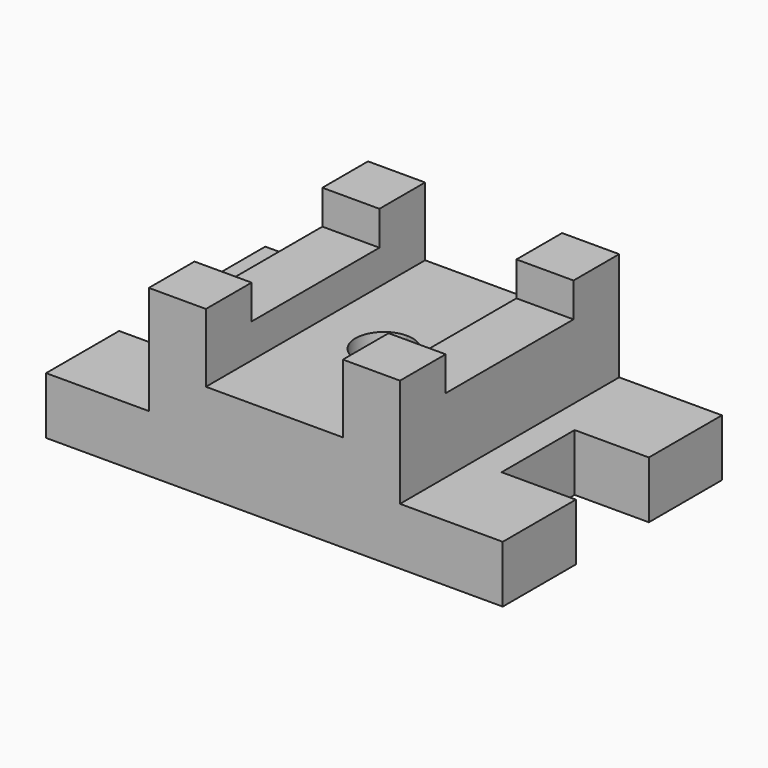
from build123d import *

# Parameters (mm, degrees)
F0_W     = 31.75
F0_H     = 88.9
F0_H_2   = 31.75
F1_DEPTH = 31.75
F2_DEPTH = 31.751
F3_DEPTH = 31.751
F4_DEPTH = 22.225
F5_DEPTH = 60.325
F6_DEPTH = 41.275
F7_SCALE = 0.5


with BuildPart() as f1:
    # F0 (on Top) → F1 (new body)
    with BuildSketch(Plane.XY):
        Polygon((-69.85, 44.45), (-69.85, 76.2), (-127, 76.2), (-127, 25.4), (-85.725, 25.4), (-85.725, -25.4), (-127, -25.4), (-127, -76.2), (-69.85, -76.2), (-69.85, -44.45), align=None)
        Polygon((-85.725, 25.4), (-127, 25.4), (-127, 0), (-127, -25.4), (-85.725, -25.4), align=None)
        with Locations((-53.975, 0)):
            Rectangle(F0_W, F0_H)
        with Locations((-53.975, 60.325)):
            Rectangle(F0_W, F0_H_2)
        with Locations((-53.975, -60.325)):
            Rectangle(F0_W, F0_H_2)
        with BuildLine():
            ThreePointArc((0, -15.875), (-15.875, 0), (0, 15.875))
            Line((0, 15.875), (0, 76.2))
            Line((0, 76.2), (-38.1, 76.2))
            Line((-38.1, 76.2), (-38.1, 44.45))
            Line((-38.1, 44.45), (-38.1, -44.45))
            Line((-38.1, -44.45), (-38.1, -76.2))
            Line((-38.1, -76.2), (0, -76.2))
            Line((0, -76.2), (0, -15.875))
        make_face()
        with BuildLine():
            Line((0, -15.875), (0, 0))
            Line((0, 0), (0, 15.875))
            ThreePointArc((0, 15.875), (-15.875, 0), (0, -15.875))
        make_face()
        with BuildLine():
            Line((0, 76.2), (0, 15.875))
            ThreePointArc((0, 15.875), (11.22532, 11.22532), (15.875, 0))
            ThreePointArc((15.875, 0), (11.22532, -11.22532), (0, -15.875))
            Line((0, -15.875), (0, -76.2))
            Line((0, -76.2), (38.1, -76.2))
            Line((38.1, -76.2), (38.1, -44.45))
            Line((38.1, -44.45), (38.1, 44.45))
            Line((38.1, 44.45), (38.1, 76.2))
            Line((38.1, 76.2), (0, 76.2))
        make_face()
        with BuildLine():
            Line((0, 15.875), (0, 0))
            Line((0, 0), (0, -15.875))
            ThreePointArc((0, -15.875), (11.22532, -11.22532), (15.875, 0))
            ThreePointArc((15.875, 0), (11.22532, 11.22532), (0, 15.875))
        make_face()
        with Locations((53.975, 0)):
            Rectangle(F0_W, F0_H)
        with Locations((53.975, 60.325)):
            Rectangle(F0_W, F0_H_2)
        with Locations((53.975, -60.325)):
            Rectangle(F0_W, F0_H_2)
        Polygon((127, 76.2), (69.85, 76.2), (69.85, 44.45), (69.85, -44.45), (69.85, -76.2), (127, -76.2), (127, -25.4), (85.725, -25.4), (85.725, 25.4), (127, 25.4), align=None)
        Polygon((127, 0), (127, 25.4), (85.725, 25.4), (85.725, -25.4), (127, -25.4), align=None)
    extrude(amount=-F1_DEPTH)

    # F0 (on Top) → F2 (cut, through all)
    with BuildSketch(Plane.XY):
        Polygon((-85.725, 25.4), (-127, 25.4), (-127, 0), (-127, -25.4), (-85.725, -25.4), align=None)
        Polygon((127, 0), (127, 25.4), (85.725, 25.4), (85.725, -25.4), (127, -25.4), align=None)
    extrude(amount=-F2_DEPTH, mode=Mode.SUBTRACT)

    # F0 (on Top) → F3 (cut, through all)
    with BuildSketch(Plane.XY):
        with BuildLine():
            Line((0, 15.875), (0, 0))
            Line((0, 0), (0, -15.875))
            ThreePointArc((0, -15.875), (11.22532, -11.22532), (15.875, 0))
            ThreePointArc((15.875, 0), (11.22532, 11.22532), (0, 15.875))
        make_face()
        with BuildLine():
            Line((0, -15.875), (0, 0))
            Line((0, 0), (0, 15.875))
            ThreePointArc((0, 15.875), (-15.875, 0), (0, -15.875))
        make_face()
    extrude(amount=-F3_DEPTH, mode=Mode.SUBTRACT)

    # F0 (on Top) → F4 (join)
    with BuildSketch(Plane.XY):
        with BuildLine():
            ThreePointArc((0, -15.875), (-15.875, 0), (0, 15.875))
            Line((0, 15.875), (0, 76.2))
            Line((0, 76.2), (-38.1, 76.2))
            Line((-38.1, 76.2), (-38.1, 44.45))
            Line((-38.1, 44.45), (-38.1, -44.45))
            Line((-38.1, -44.45), (-38.1, -76.2))
            Line((-38.1, -76.2), (0, -76.2))
            Line((0, -76.2), (0, -15.875))
        make_face()
        with BuildLine():
            Line((0, 76.2), (0, 15.875))
            ThreePointArc((0, 15.875), (11.22532, 11.22532), (15.875, 0))
            ThreePointArc((15.875, 0), (11.22532, -11.22532), (0, -15.875))
            Line((0, -15.875), (0, -76.2))
            Line((0, -76.2), (38.1, -76.2))
            Line((38.1, -76.2), (38.1, -44.45))
            Line((38.1, -44.45), (38.1, 44.45))
            Line((38.1, 44.45), (38.1, 76.2))
            Line((38.1, 76.2), (0, 76.2))
        make_face()
    extrude(amount=F4_DEPTH)

    # F0 (on Top) → F5 (join)
    with BuildSketch(Plane.XY):
        with Locations((-53.975, 60.325)):
            Rectangle(F0_W, F0_H_2)
        with Locations((-53.975, -60.325)):
            Rectangle(F0_W, F0_H_2)
        with Locations((53.975, 60.325)):
            Rectangle(F0_W, F0_H_2)
        with Locations((53.975, -60.325)):
            Rectangle(F0_W, F0_H_2)
    extrude(amount=F5_DEPTH)

    # F0 (on Top) → F6 (join)
    with BuildSketch(Plane.XY):
        with Locations((-53.975, 0)):
            Rectangle(F0_W, F0_H)
        with Locations((53.975, 0)):
            Rectangle(F0_W, F0_H)
    extrude(amount=F6_DEPTH)


with BuildPart() as f1_1:
    # F7: moved
    add(f1.part.scale(F7_SCALE))


solid = f1_1.part
